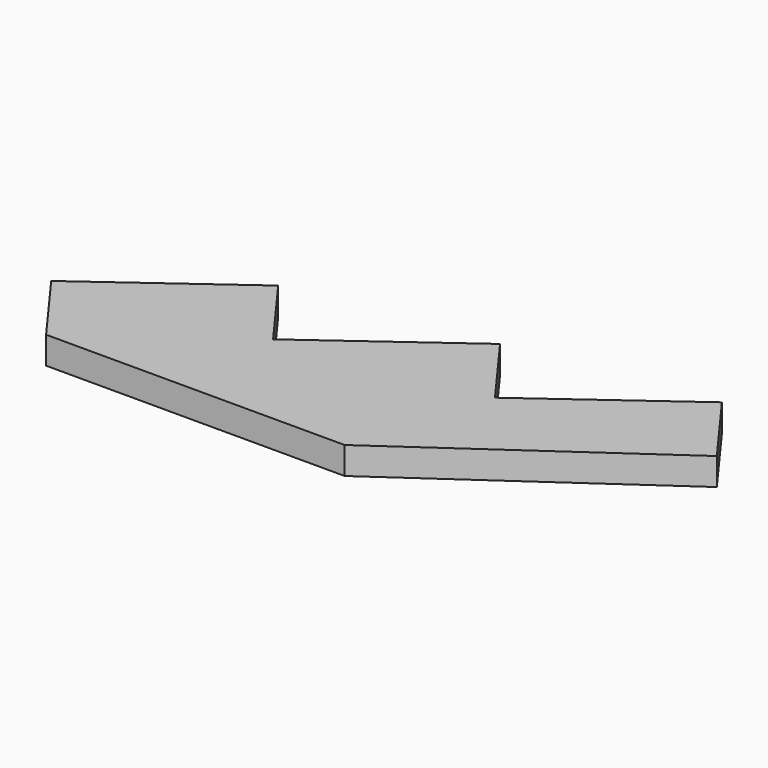
from build123d import *

# Parameters (mm, degrees)
F1_DEPTH = 38.1


# Not quite as in the source:
# - a feature of the source that left no trace in its solid (it failed there, or was rolled back) is left out


with BuildPart() as f1:
    # F0 (on Top) → F1 (new body)
    with BuildSketch(Plane.XY):
        Polygon((-1217.3470808469, 0), (-1292.2445167444, 102.564), (-1492.2443167443, -43.486), (-1417.3468808468, -146.05), (-1000.5643164725, -146.05), (-667.5526090523, 86.9720000001), (-710.694361694, 146.05), (-742.4500449497, 189.536), (-942.4498449496, 43.486), (-1017.347280847, 146.05), align=None)
    extrude(amount=F1_DEPTH)


solid = f1.part
